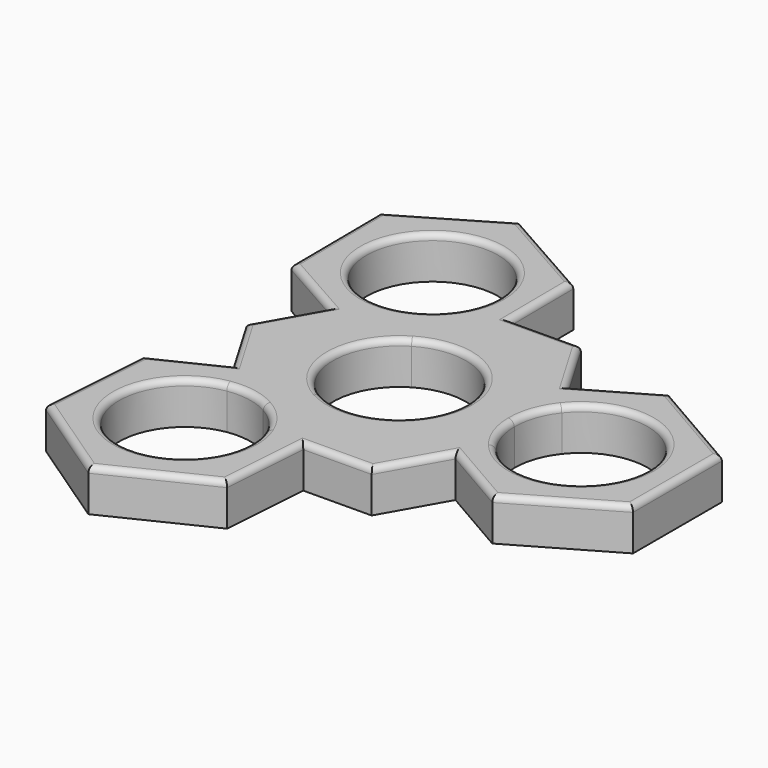
from build123d import *

# Parameters (mm, degrees)
F1_DEPTH = 7
F2_R     = 1


# Not quite as in the source:
# - a feature names something its author has since deleted; it is built from what else it names


with BuildPart() as f1:
    # F0 (on Top) → F1 (new body)
    with BuildSketch(Plane.XY):
        with BuildLine():
            Line((1.8354592313, -18.0288866684), (-6.8725484416, -12.1387655175))
            Line((-6.8725484416, -12.1387655175), (-9.3855982427, -16.577486107))
            ThreePointArc((-9.3855982427, -16.577486107), (-6.5509171288, -18.8829148956), (-4.6325469674, -21.9926214477))
            Line((-4.6325469674, -21.9926214477), (1.5568225731, -21.9404480676))
            Line((1.5568225731, -21.9404480676), (1.8354592313, -18.0288866684))
        make_face()
        with BuildLine():
            Line((-9.3855982427, -16.577486107), (-6.8725484416, -12.1387655175))
            Line((-6.8725484416, -12.1387655175), (-13.4677307337, -7.677765462))
            Line((-13.4677307337, -7.677765462), (-19.2886284671, -10.507439643))
            Line((-19.2886284671, -10.507439643), (-16.4745120744, -15.2881111147))
            ThreePointArc((-16.4745120744, -15.2881111147), (-12.8209656942, -15.3330306479), (-9.3855982427, -16.577486107))
        make_face()
        with BuildLine():
            Line((-16.4745120744, -15.2881111147), (-19.2886284671, -10.507439643))
            Line((-19.2886284671, -10.507439643), (-30.0836596385, -15.7551561274))
            Line((-30.0836596385, -15.7551561274), (-31.3963985784, -34.1836679993))
            Line((-31.3963985784, -34.1836679993), (-16.0932086134, -44.5347892056))
            Line((-16.0932086134, -44.5347892056), (0.5227202914, -36.4573985402))
            Line((0.5227202914, -36.4573985402), (1.5568225731, -21.9404480676))
            Line((1.5568225731, -21.9404480676), (-4.6325469674, -21.9926214477))
            ThreePointArc((-4.6325469674, -21.9926214477), (-4.0328593896, -24.010716983), (-3.8304696735, -26.1062773338))
            ThreePointArc((-3.8304696735, -26.1062773338), (-21.8992032586, -34.4265016183), (-16.4745120744, -15.2881111147))
        make_face()
        with BuildLine():
            Line((13.9989342061, 9.4904807568), (13.9989342061, 0.1180042183))
            Line((13.9989342061, 0.1180042183), (18.9493267735, 0.1597336241))
            ThreePointArc((18.9493267735, 0.1597336241), (19.5401979067, 3.8190137185), (21.3079276944, 7.0770178473))
            Line((21.3079276944, 7.0770178473), (18.3936825257, 12.0277898821))
            Line((18.3936825257, 12.0277898821), (13.9989342061, 9.4904807568))
        make_face()
        with BuildLine():
            Line((18.9493267735, 0.1597336241), (13.9989342061, 0.1180042183))
            Line((13.9989342061, 0.1180042183), (13.9989342061, -8.9847278573))
            Line((13.9989342061, -8.9847278573), (18.627288083, -11.656909214))
            Line((18.627288083, -11.656909214), (21.4242029382, -6.7168067341))
            ThreePointArc((21.4242029382, -6.7168067341), (19.6018014676, -3.4890656687), (18.9493267735, 0.1597336241))
        make_face()
        with BuildLine():
            Line((21.4242029382, -6.7168067341), (18.627288083, -11.656909214))
            Line((18.627288083, -11.656909214), (29.9989342061, -18.2223321643))
            Line((29.9989342061, -18.2223321643), (45.9989342061, -8.9847278573))
            Line((45.9989342061, -8.9847278573), (45.9989342061, 9.4904807568))
            Line((45.9989342061, 9.4904807568), (29.9989342061, 18.7280850638))
            Line((29.9989342061, 18.7280850638), (18.3936825257, 12.0277898821))
            Line((18.3936825257, 12.0277898821), (21.3079276944, 7.0770178473))
            ThreePointArc((21.3079276944, 7.0770178473), (33.6091196616, 10.6964898559), (41.0489342061, 0.2528764497))
            ThreePointArc((41.0489342061, 0.2528764497), (33.6970228671, -10.1599349024), (21.4242029382, -6.7168067341))
        make_face()
        with BuildLine():
            Line((-15.0627330271, 7.3788486288), (-7.1019501152, 12.0649204126))
            Line((-7.1019501152, 12.0649204126), (-9.6637249782, 16.4169095614))
            ThreePointArc((-9.6637249782, 16.4169095614), (-13.0776254326, 15.1147180995), (-16.7298953858, 15.0082140818))
            Line((-16.7298953858, 15.0082140818), (-19.5962043346, 9.9455430035))
            Line((-19.5962043346, 9.9455430035), (-15.0627330271, 7.3788486288))
        make_face()
        with BuildLine():
            Line((-9.6637249782, 16.4169095614), (-7.1019501152, 12.0649204126))
            Line((-7.1019501152, 12.0649204126), (0.8588327967, 16.7509921963))
            Line((0.8588327967, 16.7509921963), (0.8149196752, 21.9604407032))
            Line((0.8149196752, 21.9604407032), (-5.002636564, 21.9114015287))
            ThreePointArc((-5.002636564, 21.9114015287), (-6.868311211, 18.7697973162), (-9.6637249782, 16.4169095614))
        make_face()
        with BuildLine():
            Line((-5.002636564, 21.9114015287), (0.8149196752, 21.9604407032))
            Line((0.8149196752, 21.9604407032), (0.7031012913, 35.2255444515))
            Line((0.7031012913, 35.2255444515), (-15.374196038, 44.3279531393))
            Line((-15.374196038, 44.3279531393), (-31.2957618618, 34.9558095718))
            Line((-31.2957618618, 34.9558095718), (-31.1400303564, 16.4812573166))
            Line((-31.1400303564, 16.4812573166), (-19.5962043346, 9.9455430035))
            Line((-19.5962043346, 9.9455430035), (-16.7298953858, 15.0082140818))
            ThreePointArc((-16.7298953858, 15.0082140818), (-22.4070781735, 34.1133242446), (-4.2684645325, 25.8534008841))
            ThreePointArc((-4.2684645325, 25.8534008841), (-4.4535721444, 23.8485088989), (-5.002636564, 21.9114015287))
        make_face()
        with BuildLine():
            ThreePointArc((-5.6054677695, 9.5226693256), (5.4441396631, 9.6158121513), (11.0496074326, 0.0931428257))
            Line((11.0496074326, 0.0931428257), (13.9989342061, 0.1180042183))
            Line((13.9989342061, 0.1180042183), (13.9989342061, 9.4904807568))
            Line((13.9989342061, 9.4904807568), (18.3936825257, 12.0277898821))
            Line((18.3936825257, 12.0277898821), (12.4889549437, 22.0588471523))
            Line((12.4889549437, 22.0588471523), (0.8149196752, 21.9604407032))
            Line((0.8149196752, 21.9604407032), (0.8588327967, 16.7509921963))
            Line((0.8588327967, 16.7509921963), (-7.1019501152, 12.0649204126))
            Line((-7.1019501152, 12.0649204126), (-5.6054677695, 9.5226693256))
        make_face()
        with BuildLine():
            Line((-6.8725484416, -12.1387655175), (-5.4441396631, -9.6158121513))
            ThreePointArc((-5.4441396631, -9.6158121513), (-11.0496074326, -0.0931428257), (-5.6054677695, 9.5226693256))
            Line((-5.6054677695, 9.5226693256), (-7.1019501152, 12.0649204126))
            Line((-7.1019501152, 12.0649204126), (-15.0627330271, 7.3788486288))
            Line((-15.0627330271, 7.3788486288), (-19.5962043346, 9.9455430035))
            Line((-19.5962043346, 9.9455430035), (-25.3479994839, -0.2136713282))
            Line((-25.3479994839, -0.2136713282), (-19.2886284671, -10.507439643))
            Line((-19.2886284671, -10.507439643), (-13.4677307337, -7.677765462))
            Line((-13.4677307337, -7.677765462), (-6.8725484416, -12.1387655175))
        make_face()
        with BuildLine():
            ThreePointArc((11.0496074326, 0.0931428257), (11.0499018577, 0.0465718265), (11.05, 0))
            ThreePointArc((11.05, 0), (5.5652833137, -9.5462098049), (-5.4441396631, -9.6158121513))
            Line((-5.4441396631, -9.6158121513), (-6.8725484416, -12.1387655175))
            Line((-6.8725484416, -12.1387655175), (1.8354592313, -18.0288866684))
            Line((1.8354592313, -18.0288866684), (1.5568225731, -21.9404480676))
            Line((1.5568225731, -21.9404480676), (12.8590445403, -21.8451758241))
            Line((12.8590445403, -21.8451758241), (18.627288083, -11.656909214))
            Line((18.627288083, -11.656909214), (13.9989342061, -8.9847278573))
            Line((13.9989342061, -8.9847278573), (13.9989342061, 0.1180042183))
            Line((13.9989342061, 0.1180042183), (11.0496074326, 0.0931428257))
        make_face()
    extrude(amount=F1_DEPTH)

    # F2
    f2_edges = [f1.edges().sort_by_distance(p)[0] for p in [
        (-23.744804, -39.359229, 7),
        (-7.785244, -40.496094, 7),
        (1.039771, -29.198923, 7),
        (7.207934, -21.892812, 7),
        (15.743166, -16.751043, 7),
        (24.313111, -14.939621, 7),
        (37.998934, -13.60353, 7),
        (45.998934, 0.252876, 7),
        (37.998934, 14.109283, 7),
        (24.196308, 15.377937, 7),
        (15.441319, 17.043319, 7),
        (6.651937, 22.009644, 7),
        (0.75901, 28.592993, 7),
        (-7.335547, 39.776749, 7),
        (-23.334979, 39.641881, 7),
        (-31.217896, 25.718533, 7),
        (-25.368117, 13.2134, 7),
        (-22.472102, 4.865936, 7),
        (-22.318314, -5.360555, 7),
        (-24.686144, -13.131298, 7),
        (-30.740029, -24.969412, 7),
        (-13.086427, -36.924444, 7),
        (38.689941, -6.571265, 7),
        (-13.707034, 36.698588, 7),
        (-11.049607, -0.093143, 7),
    ]]
    fillet(f2_edges, radius=F2_R)


solid = f1.part
